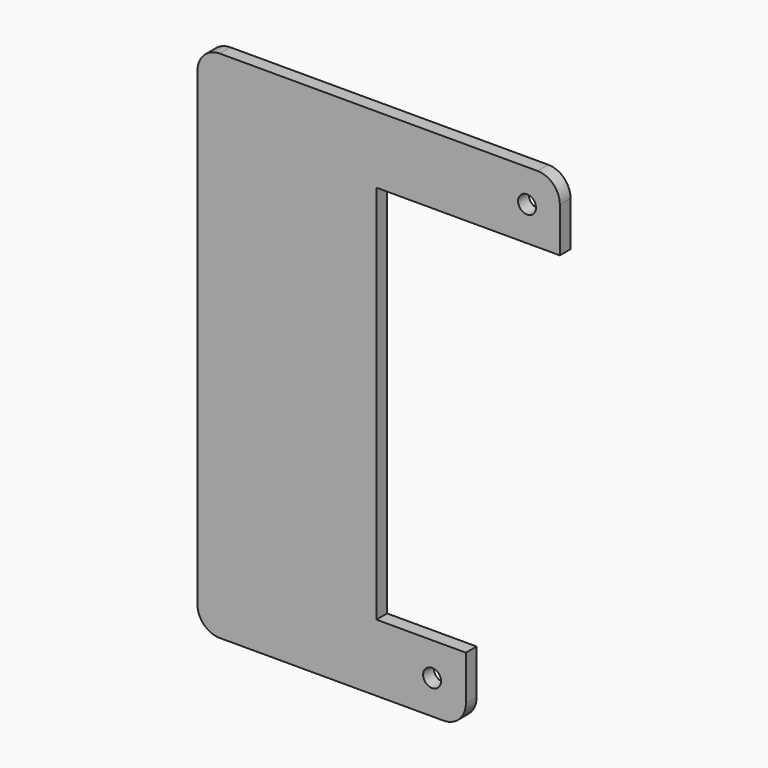
from build123d import *

# Parameters (mm, degrees)
F0_R     = 2
F1_DEPTH = 3
F2_R     = 5


# Not quite as in the source:
# - a feature names something its author has since deleted; it is built from what else it names


with BuildPart() as f1:
    # F0 (on Front) → F1 (new body)
    with BuildSketch(Plane.XZ):
        Polygon((-81, 51.5256257355), (-81, -63.4743742645), (-21, -63.4743742645), (-21, -48.4743742645), (-41, -48.4743742645), (-41, -15.9743742645), (-41, 4.0256257355), (-41, 36.5256257355), (0, 36.5256257355), (0, 51.5256257355), align=None)
        with Locations((-28.5549983382, -55.90621382)):
            Circle(F0_R, mode=Mode.SUBTRACT)
        with Locations((-7.3309438303, 44.1784150898)):
            Circle(F0_R, mode=Mode.SUBTRACT)
    extrude(amount=F1_DEPTH)

    # F2
    f2_edges = [f1.edges().sort_by_distance(p)[0] for p in [
        (-81, -1.5, 51.525626),
        (-81, -1.5, -63.474374),
        (0, -1.5, 51.525626),
        (-21, -1.5, -63.474374),
    ]]
    fillet(f2_edges, radius=F2_R)


solid = f1.part
